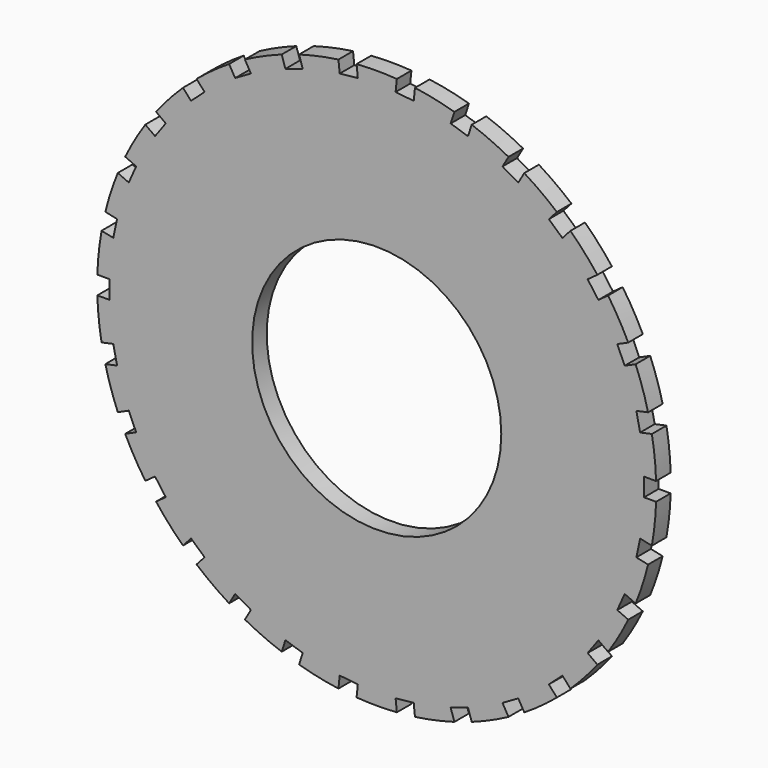
from build123d import *

# Parameters (mm, degrees)
F0_R            = 46
F0_R_2          = 20.5
F1_DEPTH        = 3
F2_W            = 2
F2_H            = 3
F3_DEPTH        = 3
F3_COPIES_COUNT = 30


# Not quite as in the source:
# - a pattern or mirror of a feature is missing from the dataset's text; its kind, count and spacing are read off the source's solid


with BuildPart() as f1:
    # F0 (on Front) → F1 (new body)
    with BuildSketch(Plane.XZ):
        Circle(F0_R)
        Circle(F0_R_2, mode=Mode.SUBTRACT)
    extrude(amount=F1_DEPTH)

    # F2 (on Front) → F3 (cut)
    with BuildSketch(Plane.XZ):
        with Locations((-45, 0)):
            Rectangle(F2_W, F2_H)
    f3 = extrude(amount=F3_DEPTH, mode=Mode.SUBTRACT)

    # F3_copies: F3 ×30 about axis
    f3_copies_axis = Axis((0, 0, 0), (0, 1, 0))
    for i in range(1, F3_COPIES_COUNT):
        add(f3.rotate(f3_copies_axis, i * 360 / F3_COPIES_COUNT), mode=Mode.SUBTRACT)


solid = f1.part
